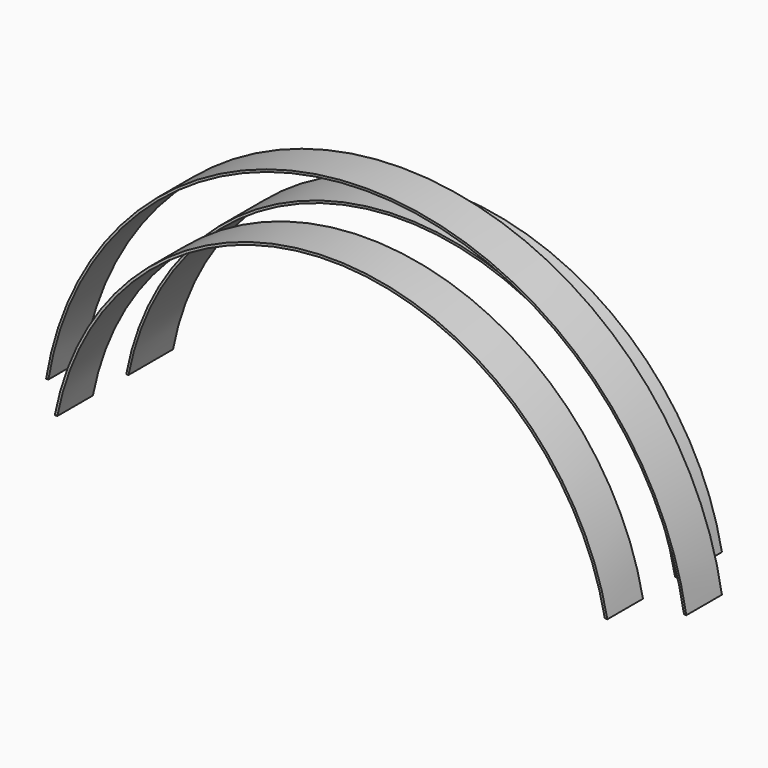
from build123d import *

# Parameters (mm, degrees)
F1_DEPTH = 12700
F3_DEPTH = 10160
F5_DEPTH = 10160


# Not quite as in the source:
# - the program builds the solid bodies; features that only make, move or delete a surface that nothing else refers to are left out


with BuildPart() as f1:
    # F0 (on Front) → F1 (new body)
    with BuildSketch(Plane.XZ):
        with BuildLine():
            ThreePointArc((18.0655783815, 94.7577951073), (62385.5195391376, 51655.2985756552), (124752.9734998938, 94.7577951073))
            Line((124752.9734998938, 94.7577951073), (125270.1242021943, 94.7577951073))
            ThreePointArc((125270.1242021943, 94.7577951073), (62385.5195391376, 52163.2995605469), (-499.0851239191, 94.7577951073))
            Line((-499.085123919, 94.7577951073), (18.0655783815, 94.7577951073))
        make_face()
    extrude(amount=F1_DEPTH)


with BuildPart() as f3:
    # F2 (on face) → F3 (new body)
    with BuildSketch(Plane.XZ.offset(12700)):
        with BuildLine():
            Line((134915.2767422943, 0), (135430.1242021946, 0))
            ThreePointArc((135430.1242021946, 0), (62385.5195391377, 62031.7013759603), (-10659.0851239193, 0))
            Line((-10659.0851239193, 0), (-10144.237664019, 0))
            ThreePointArc((-10144.2376640191, 0), (62385.5195391376, 61523.7007141114), (134915.2767422944, 0))
        make_face()
    extrude(amount=F3_DEPTH)


with BuildPart() as f5:
    # F4 (on face) → F5 (new body)
    with BuildSketch(Plane.XZ.offset(22860)):
        with BuildLine():
            ThreePointArc((20.6717815327, 106.2507860158), (62498.1346130371, 51555.2062289571), (124975.5974445415, 106.2507860157))
            Line((124975.5974445415, 106.2507860157), (125544.8747328501, 106.2507860157))
            ThreePointArc((125544.8747328501, 106.2507860157), (62498.1346130371, 52114.0060424805), (-548.6055067759, 106.2507860157))
            Line((-548.6055067759, 106.2507860157), (20.6717815327, 106.2507860157))
        make_face()
    extrude(amount=F5_DEPTH)


solid = Compound([f1.part, f3.part, f5.part])
